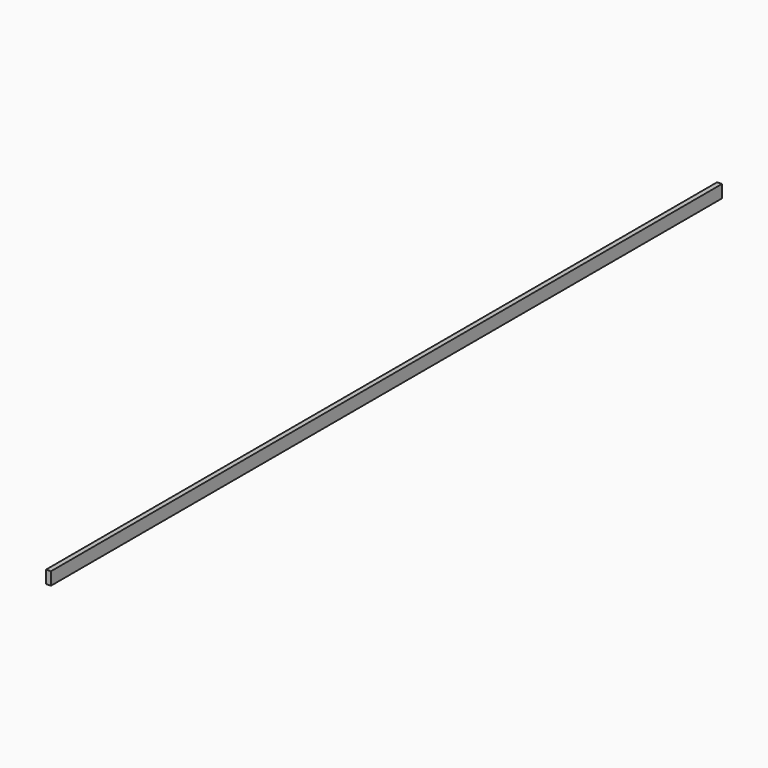
from build123d import *

# Parameters (mm, degrees)
F0_W     = 19.05
F0_H     = 50.8
F1_DEPTH = 3343.275


# Not quite as in the source:
# - a length typed as a fraction of an inch, garbled in the dataset ("3 / 203.2 mm" for 3/8 in), is restored


with BuildPart() as f1:
    # F0 (on Front) → F1 (new body)
    with BuildSketch(Plane.XZ):
        with Locations((9.525, -25.4)):
            Rectangle(F0_W, F0_H)
    extrude(amount=-F1_DEPTH)


solid = f1.part
